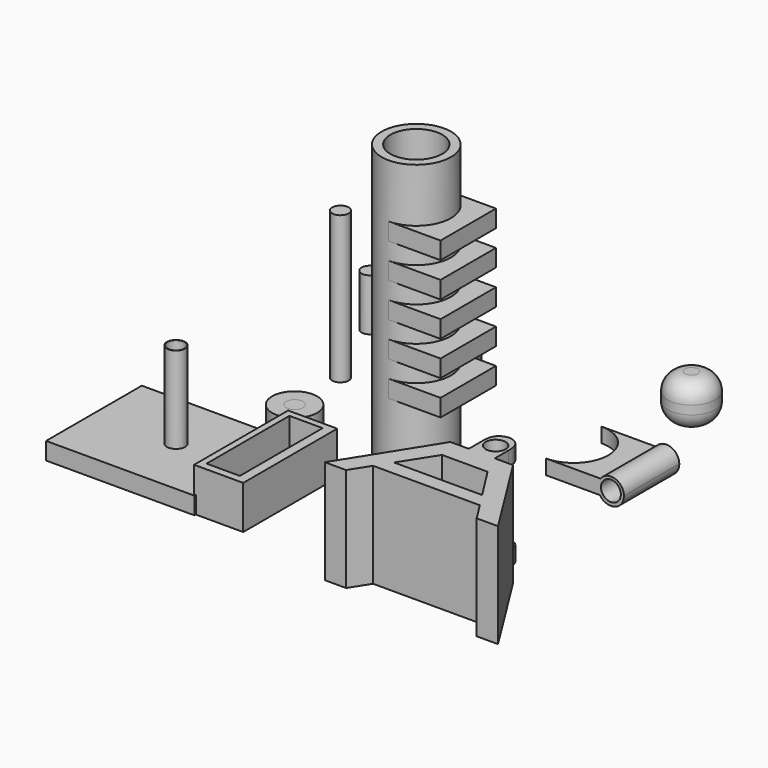
from build123d import *

# Parameters (mm, degrees)
F0_R         = 10.16
F0_R_2       = 7.62
F1_DEPTH     = 86.36
F3_R         = 2.794
F4_DEPTH     = 7.62
F5_R         = 2.413
F6_DEPTH     = 15.24
F7_W         = 43.5428619385
F7_H         = 35.1064288989
F8_DEPTH     = 5.08
F9_W         = 14.4067853689
F9_H         = 34.4903981313
F10_DEPTH    = 12.7
F11_R        = 2.667
F12_DEPTH    = 25.4
F13_R        = 2.54
F14_DEPTH    = 10.16
F15_W        = 9.7603034228
F15_H        = 30.3600495681
F16_DEPTH    = 10.16
F17_R        = 2.413
F18_DEPTH    = 43.18
F19_R        = 6.9088
F20_DEPTH    = 5.08
F21_R        = 2.54
F22_DEPTH    = 3.81
F23_R        = 6.096
F24_DEPTH    = 19.05
F25_R        = 5.08
F26_SIZE     = 5.08
F27_R        = 15.24
F28_R        = 2.54
F28_R_2      = 1.016
F29_DEPTH    = 5.08
F30_DEPTH    = 5.08
F31_R        = 6.604
F31_R_2      = 2.4638
F32_DEPTH    = 6.35
F34_W        = 20.3210590407
F34_H        = 2.54
F35_DEPTH    = 15.24
F2_R         = 7.62
F36_DEPTH    = 88.9
F37_DEPTH    = 0.635
F0_R_3       = 2.794
F38_DEPTH    = 5.08
F40_DEPTH    = 4.318
F42_DEPTH    = 20.32
F44_DEPTH    = 30.48
F45_W        = 7.62
F45_H        = 4.318
F46_DEPTH    = 10.16
F48_DEPTH    = 35.56
F49_T1_DEPTH = 29.718
F49_T3_DEPTH = 29.718
F50_R        = 6.985
F51_DEPTH    = 12.7
F52_R        = 5.08


# Not quite as in the source:
# - a fillet or chamfer that OpenCascade refuses, or shapes differently, is made with other operations: its cross-section is extruded or revolved along the edge and cut away or added
# - a feature names something its author has since deleted; it is built from what else it names


with BuildPart() as f1:
    # F0 (on Top) → F1 (new body)
    with BuildSketch(Plane.XY):
        Circle(F0_R)
        Circle(F0_R_2, mode=Mode.SUBTRACT)
    extrude(amount=F1_DEPTH)

    # F3 (on face) → F4 (cut)
    with BuildSketch(Plane(origin=(0, 0, 0), x_dir=(1, 0, 0), z_dir=(0, 0, -1))):
        Circle(F3_R)
    extrude(amount=-F4_DEPTH, mode=Mode.SUBTRACT)

    # F34 (on Right) → F35 (join)
    with BuildSketch(Plane.YZ):
        with Locations((0.0005946495, 69.3213942552)):
            Rectangle(F34_W, F34_H)
        with Locations((0.0005946495, 66.7813942552)):
            Rectangle(F34_W, F34_H)
        with Locations((0.0005946495, 59.1613942552)):
            Rectangle(F34_W, F34_H)
        with Locations((0.0005946495, 56.6213942552)):
            Rectangle(F34_W, F34_H)
        Polygon((10.1611241698, 50.2713942552), (-10.1599348709, 50.2713942552), (-10.1599348709, 48.2687056065), (-10.1599348709, 47.7313942552), (10.1611241698, 47.7313942552), align=None)
        with Locations((0.0005946495, 46.4613942552)):
            Rectangle(F34_W, F34_H)
        with Locations((0.0005946495, 38.8413942552)):
            Rectangle(F34_W, F34_H)
        with Locations((0.0005946495, 36.3013942552)):
            Rectangle(F34_W, F34_H)
        with Locations((0.0005946495, 28.6813942552)):
            Rectangle(F34_W, F34_H)
        with Locations((0.0005946495, 26.1413942552)):
            Rectangle(F34_W, F34_H)
    extrude(amount=F35_DEPTH)

    # F2 (on face) → F36 (cut)
    with BuildSketch(Plane.XY.offset(86.36)):
        Circle(F2_R)
    extrude(amount=-F36_DEPTH, mode=Mode.SUBTRACT)

    # F0 (on Top) → F38 (join)
    with BuildSketch(Plane.XY):
        Circle(F0_R_2)
        Circle(F0_R_3, mode=Mode.SUBTRACT)
    extrude(amount=F38_DEPTH)


with BuildPart() as f6:
    # F5 (on Top) → F6 (new body)
    with BuildSketch(Plane.XY):
        with Locations((-54.5346215367, 51.1315390468)):
            Circle(F5_R)
    extrude(amount=F6_DEPTH)


with BuildPart() as f8:
    # F7 (on Top) → F8 (new body)
    with BuildSketch(Plane.XY):
        with Locations((-50.0742867589, -28.4389290027)):
            Rectangle(F7_W, F7_H)
    extrude(amount=F8_DEPTH)

    # F9 (on Top) → F10 (join)
    with BuildSketch(Plane.XY):
        with Locations((-21.6104313731, -28.2431771047)):
            Rectangle(F9_W, F9_H)
    extrude(amount=F10_DEPTH)

    # F11 (on face) → F12 (join)
    with BuildSketch(Plane.XY.offset(5.08)):
        with Locations((-47.7637946606, -28.4398160875)):
            Circle(F11_R)
    extrude(amount=F12_DEPTH)

    # F13 (on face) → F14 (cut)
    with BuildSketch(Plane.XY.offset(30.48)):
        with Locations((-47.7637946606, -28.4398160875)):
            Circle(F13_R)
    extrude(amount=-F14_DEPTH, mode=Mode.SUBTRACT)

    # F15 (on face) → F16 (cut)
    with BuildSketch(Plane.XY.offset(12.7)):
        with Locations((-22.0615947619, -28.0654546805)):
            Rectangle(F15_W, F15_H)
    extrude(amount=-F16_DEPTH, mode=Mode.SUBTRACT)


with BuildPart() as f18:
    # F17 (on Top) → F18 (new body)
    with BuildSketch(Plane.XY):
        with Locations((-44.9035726488, 28.3028576523)):
            Circle(F17_R)
    extrude(amount=F18_DEPTH)


with BuildPart() as f20:
    # F19 (on Top) → F20 (new body)
    with BuildSketch(Plane.XY):
        with Locations((-20.6828564405, 16.6007149965)):
            Circle(F19_R)
    extrude(amount=F20_DEPTH)

    # F21 (on face) → F22 (cut)
    with BuildSketch(Plane.XY.offset(5.08)):
        with Locations((-20.6828564405, 16.6007149965)):
            Circle(F21_R)
    extrude(amount=-F22_DEPTH, mode=Mode.SUBTRACT)


with BuildPart() as f24:
    # F23 (on Top) → F24 (new body)
    with BuildSketch(Plane.XY):
        with Locations((-18.8286863267, 37.8593802452)):
            Circle(F23_R)
    extrude(amount=F24_DEPTH)

    # F25
    f25_edges = [f24.edges().sort_by_distance(p)[0] for p in [
        (-24.924686, 37.85938, 19.05),
    ]]
    fillet(f25_edges, radius=F25_R)

    # F26
    f26_edges = [f24.edges().sort_by_distance(p)[0] for p in [
        (-24.924686, 37.85938, 0),
    ]]
    chamfer(f26_edges, length=F26_SIZE)

    # F27
    f27_edges = [f24.edges().sort_by_distance(p)[0] for p in [
        (-12.732686, 37.85938, 9.525),
        (-24.924686, 37.85938, 5.08),
        (-24.924686, 37.85938, 13.97),
    ]]
    fillet(f27_edges, radius=F27_R)

    # F28 (on face) → F29 (cut)
    with BuildSketch(Plane(origin=(0, 0, 0), x_dir=(1, 0, 0), z_dir=(0, 0, -1))):
        with Locations((-18.8286863267, -37.8593802452)):
            Circle(F28_R)
        with Locations((-18.8286863267, -37.8593802452)):
            Circle(F28_R_2, mode=Mode.SUBTRACT)
    extrude(amount=-F29_DEPTH, mode=Mode.SUBTRACT)

    # F30 (cut): a face of the model
    f30_faces = [f24.faces().sort_by_distance(p)[0] for p in [
        (-18.8286863267, 37.8593802452, 0),
    ]]
    extrude(f30_faces, amount=-F30_DEPTH, mode=Mode.SUBTRACT)


with BuildPart() as f32:
    # F31 (on Top) → F32 (new body)
    with BuildSketch(Plane.XY):
        with Locations((-44.7303764522, 11.2661803141)):
            Circle(F31_R)
        with Locations((-44.7303764522, 11.2661803141)):
            Circle(F31_R_2, mode=Mode.SUBTRACT)
    extrude(amount=-F32_DEPTH)


with BuildPart() as f37:
    # F31 (on Top) → F37 (new body)
    with BuildSketch(Plane.XY):
        with Locations((-44.7303764522, 11.2661803141)):
            Circle(F31_R_2)
    extrude(amount=-F37_DEPTH)


with BuildPart() as f40:
    # F39 (on Top) → F40 (new body)
    with BuildSketch(Plane.XY):
        with BuildLine():
            Line((37.3759008944, 40.215914942), (22.1359008944, 40.215914942))
            ThreePointArc((22.1359008944, 40.215914942), (29.3201057913, 37.2401198389), (32.2959008944, 30.055914942))
            Line((32.2959008944, 30.055914942), (37.3759008944, 30.055914942))
            Line((37.3759008944, 30.055914942), (37.3759008944, 40.215914942))
        make_face()
        with BuildLine():
            ThreePointArc((32.2959008944, 30.055914942), (29.3201057913, 22.8717100452), (22.1359008944, 19.895914942))
            Line((22.1359008944, 19.895914942), (37.3759008944, 19.895914942))
            Line((37.3759008944, 19.895914942), (37.3759008944, 30.055914942))
            Line((37.3759008944, 30.055914942), (32.2959008944, 30.055914942))
        make_face()
    extrude(amount=F40_DEPTH)

    # F41 (on face) → F42 (join)
    with BuildSketch(Plane.XZ.offset(-19.895914942)):
        with BuildLine():
            ThreePointArc((38.2649008944, 2.159), (41.1859008944, 5.08), (44.1069008944, 2.159))
            Line((44.1069008944, 2.159), (44.9959008944, 2.159))
            ThreePointArc((44.9959008944, 2.159), (42.3276792685, 5.6903392456), (38.1197761674, 4.318))
            ThreePointArc((38.1197761674, 4.318), (37.5823480551, 3.2955191166), (37.3759008944, 2.159))
            Line((37.3759008944, 2.159), (38.2649008944, 2.159))
        make_face()
        with BuildLine():
            Line((44.9959008944, 2.159), (44.1069008944, 2.159))
            ThreePointArc((44.1069008944, 2.159), (41.1859008944, -0.762), (38.2649008944, 2.159))
            Line((38.2649008944, 2.159), (37.3759008944, 2.159))
            ThreePointArc((37.3759008944, 2.159), (37.5133220868, 1.034465592), (37.9752129372, 0))
            ThreePointArc((37.9752129372, 0), (42.2558934311, -1.604247956), (44.9973494369, 2.053928634))
            ThreePointArc((44.9973494369, 2.053928634), (44.9969872841, 2.1064693093), (44.9959008944, 2.159))
        make_face()
        with BuildLine():
            Line((37.3759008944, 0), (37.9752129372, 0))
            ThreePointArc((37.9752129372, 0), (37.5428217008, 0.9336099377), (37.3759008944, 1.948857268))
            Line((37.3759008944, 1.948857268), (37.3759008944, 0))
        make_face()
        with BuildLine():
            ThreePointArc((37.3759008944, 2.159), (37.5823480551, 3.2955191166), (38.1197761674, 4.318))
            Line((38.1197761674, 4.318), (37.3759008944, 4.318))
            Line((37.3759008944, 4.318), (37.3759008944, 2.159))
        make_face()
    extrude(amount=-F42_DEPTH)


with BuildPart() as f44:
    # F43 (on Top) → F44 (new body)
    with BuildSketch(Plane.XY):
        Polygon((27.5866982771, -42.6542611828), (24.8543604423, -46.9377562391), (56.1718608992, -46.9377562391), (53.440914158, -42.6542611828), align=None)
        Polygon((31.31670226, -26.6319075943), (15.11150226, -52.4536147714), (21.3359277695, -52.4536147714), (24.8543604423, -46.9377562391), (27.5866982771, -42.6542611828), (33.8374687846, -32.8549075943), (47.193326056, -32.8549075943), (53.440914158, -42.6542611828), (56.1718608992, -46.9377562391), (59.68850226, -52.4536147714), (65.91150226, -52.4536147714), (49.7167550109, -26.6319075943), align=None)
    extrude(amount=F44_DEPTH)

    # F45 (on face) → F46 (join)
    with BuildSketch(Plane(origin=(0, -26.6319075943, 0), x_dir=(-1, 0, 0), z_dir=(0, 1, 0))):
        Polygon((-36.7067286354, 30.48), (-40.5167286354, 30.48), (-44.3267286354, 30.48), (-44.3267286354, 26.162), (-36.7067286354, 26.162), align=None)
        with Locations((-40.5167286354, 2.159)):
            Rectangle(F45_W, F45_H)
    extrude(amount=F46_DEPTH)

    # F47 (on face) → F48 (cut)
    with BuildSketch(Plane(origin=(0, 0, 0), x_dir=(1, 0, 0), z_dir=(0, 0, -1))):
        with BuildLine():
            ThreePointArc((43.4377286354, 21.5519075943), (40.5167286354, 24.4729075943), (37.5957286354, 21.5519075943))
            ThreePointArc((37.5957286354, 21.5519075943), (40.5167286354, 18.6309075943), (43.4377286354, 21.5519075943))
        make_face()
    extrude(amount=-F48_DEPTH, mode=Mode.SUBTRACT)

    # F49: fillet of radius 5.08 on 4 edges, made by hand

    # F49_s2 → F49_t1 (cut)
    with BuildSketch(Plane.XY.offset(-12.7)):
        with BuildLine():
            add(Edge.make_bspline(
                [(44.3267286354, -21.5519075943), (44.3267286354, -16.4719075943), (39.2467286354, -16.4719075943)],
                knots=[0, 0, 0, 1, 1, 1], degree=2, weights=[1, 1.1459227468, 1]))
            Line((39.2467286354, -16.4719075943), (44.3267286354, -16.4719075943))
            Line((44.3267286354, -16.4719075943), (44.3267286354, -21.5519075943))
        make_face()
        with BuildLine():
            add(Edge.make_bspline(
                [(36.7067286354, -21.5519075943), (36.7067286354, -16.4719075943), (41.7867286354, -16.4719075943)],
                knots=[0, 0, 0, 1, 1, 1], degree=2, weights=[1, 1.1459227468, 1]))
            Line((41.7867286354, -16.4719075943), (36.7067286354, -16.4719075943))
            Line((36.7067286354, -16.4719075943), (36.7067286354, -21.5519075943))
        make_face()
    extrude(amount=F49_T1_DEPTH, mode=Mode.SUBTRACT)

    # F49_s4 → F49_t3 (cut)
    with BuildSketch(Plane.XY.offset(13.462)):
        with BuildLine():
            add(Edge.make_bspline(
                [(36.7067286354, -21.5519075943), (36.7067286354, -16.4719075943), (41.7867286354, -16.4719075943)],
                knots=[0, 0, 0, 1, 1, 1], degree=2, weights=[1, 1.1459227468, 1]))
            Line((41.7867286354, -16.4719075943), (36.7067286354, -16.4719075943))
            Line((36.7067286354, -16.4719075943), (36.7067286354, -21.5519075943))
        make_face()
        with BuildLine():
            add(Edge.make_bspline(
                [(44.3267286354, -21.5519075943), (44.3267286354, -16.4719075943), (39.2467286354, -16.4719075943)],
                knots=[0, 0, 0, 1, 1, 1], degree=2, weights=[1, 1.1459227468, 1]))
            Line((39.2467286354, -16.4719075943), (44.3267286354, -16.4719075943))
            Line((44.3267286354, -16.4719075943), (44.3267286354, -21.5519075943))
        make_face()
    extrude(amount=F49_T3_DEPTH, mode=Mode.SUBTRACT)


with BuildPart() as f51:
    # F50 (on Top) → F51 (new body)
    with BuildSketch(Plane.XY):
        with Locations((31.2253832817, 61.900164932)):
            Circle(F50_R)
    extrude(amount=F51_DEPTH)

    # F52
    f52_edges = [f51.edges().sort_by_distance(p)[0] for p in [
        (24.240383, 61.900165, 12.7),
        (38.210383, 61.900165, 6.35),
        (24.240383, 61.900165, 0),
    ]]
    fillet(f52_edges, radius=F52_R)


solid = Compound([f1.part, f6.part, f8.part, f18.part, f24.part, f32.part, f37.part, f40.part, f44.part, f51.part])
